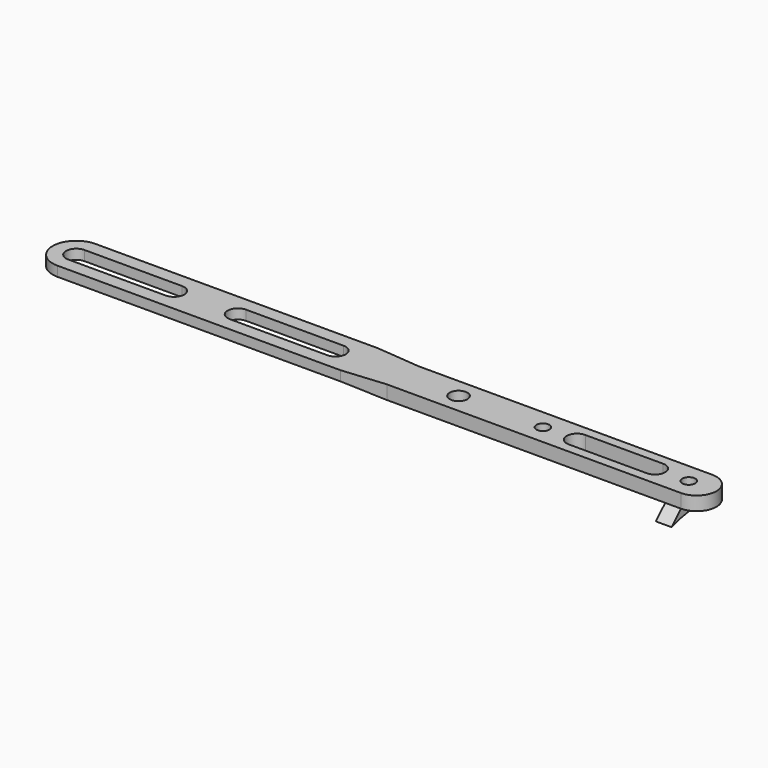
from build123d import *

# Parameters (mm, degrees)
F0_R      = 1.65
F1_DEPTH  = 3.5
F3_DEPTH  = 6
F6_DEPTH  = 2
F9_DEPTH  = 1.75
F11_D     = 4.5
F11_DEPTH = 52.4
F11_TIP   = 1.3519363928


# Not quite as in the source:
# - a feature names something its author has since deleted; it is built from what else it names


with BuildPart() as f1:
    # F0 (on Top) → F1 (new body)
    with BuildSketch(Plane.XY):
        with BuildLine():
            Line((0, 6), (-71.8000936901, 6))
            ThreePointArc((-71.8000936901, 6), (-77.8000936901, 0), (-71.8000936901, -6))
            Line((-71.8000936901, -6), (0, -6))
            Line((0, -6), (11, -5))
            Line((11, -5), (85.6788979987, -5))
            ThreePointArc((85.6788979733, -4.9999999898), (90.6788979733, 3.56e-08), (85.6788979225, 5.0000000102))
            Line((85.6788979479, 5.0000000203), (11, 4.9999992617))
            Line((11, 4.9999992617), (0, 6))
        make_face()
        with Locations((46.6788982548, -0.0513669582)):
            Circle(F0_R, mode=Mode.SUBTRACT)
        with BuildLine():
            ThreePointArc((75.0788576977, 2.5999999997), (77.6788979986, 1.85129e-05), (75.0788947235, -2.6))
            Line((75.0788947235, -2.6), (55.290283107, -2.5999750728))
            ThreePointArc((55.290283107, -2.5999750728), (55.2788947235, -2.6), (55.2675063401, -2.5999750441))
            ThreePointArc((55.2675063401, -2.5999750441), (52.6790245248, 0.02564995), (55.3188054687, 2.5996937115))
            Line((55.3188054687, 2.5996937115), (75.0788576977, 2.5999999997))
        make_face(mode=Mode.SUBTRACT)
        with BuildLine():
            ThreePointArc((-71.8000936901, -2.6), (-74.4000936901, 0), (-71.8000936901, 2.6))
            Line((-71.8000936901, 2.6), (-47.0008072172, 2.6))
            ThreePointArc((-47.0008072172, 2.6), (-44.4008072172, 0), (-47.0008072172, -2.6))
            Line((-47.0008072172, -2.6), (-71.8000936901, -2.6))
        make_face(mode=Mode.SUBTRACT)
        with BuildLine():
            ThreePointArc((-30.8000002499, -2.6), (-33.4000002499, 0), (-30.8000002499, 2.6))
            Line((-30.8000002499, 2.6), (-6.00000025, 2.6))
            ThreePointArc((-6.00000025, 2.6), (-5.9984911006, 2.599999562), (-5.9969819517, 2.5999982481))
            ThreePointArc((-5.9969819517, 2.5999982481), (-3.400000688, -0.0015091494), (-6.00000025, -2.6))
            Line((-6.00000025, -2.6), (-30.8000002499, -2.6))
        make_face(mode=Mode.SUBTRACT)
        with Locations((83.6788979987, 0)):
            Circle(F0_R, mode=Mode.SUBTRACT)
    extrude(amount=F1_DEPTH)

    # F2 (on Front) → F3 (cut, symmetric)
    with BuildSketch(Plane.XZ):
        Polygon((-80.4351404223, 1), (-80.4351404223, 0), (11, 0), (0, 1), align=None)
    extrude(amount=F3_DEPTH, both=True, mode=Mode.SUBTRACT)

    # F5 (on face) → F6 (join, symmetric)
    with BuildSketch(Plane.YZ.offset(83.6788979987)):
        Polygon((-5.7500000356, -0.75), (5.7500000356, -0.75), (5.0000000356, 0), (-5.0000000356, 0), align=None)
        with BuildLine():
            ThreePointArc((-7.9520996302, -2.9520995947), (0, -1.5), (7.9520996302, -2.9520995946))
            Line((7.9520996302, -2.9520995946), (5.7500000356, -0.75))
            Line((5.7500000356, -0.75), (-5.7500000356, -0.75))
            Line((-5.7500000356, -0.75), (-7.9520996302, -2.9520995946))
        make_face()
    extrude(amount=F6_DEPTH, both=True)

    # F9 (cut): a face of the model
    f9_faces = [f1.faces().sort_by_distance(p)[0] for p in [
        (83.6788979987, 0, 0),
    ]]
    extrude(f9_faces, amount=-F9_DEPTH, mode=Mode.SUBTRACT)

    # F11
    with Locations(Plane.XY.offset(3.5)):
        with Locations((25.2248030156, 0)):
            Hole(F11_D / 2, depth=F11_DEPTH)
            with Locations((0, 0, -(F11_DEPTH + F11_TIP / 2))):  # 118° drill point
                Cone(0, F11_D / 2, F11_TIP, mode=Mode.SUBTRACT)


solid = f1.part
